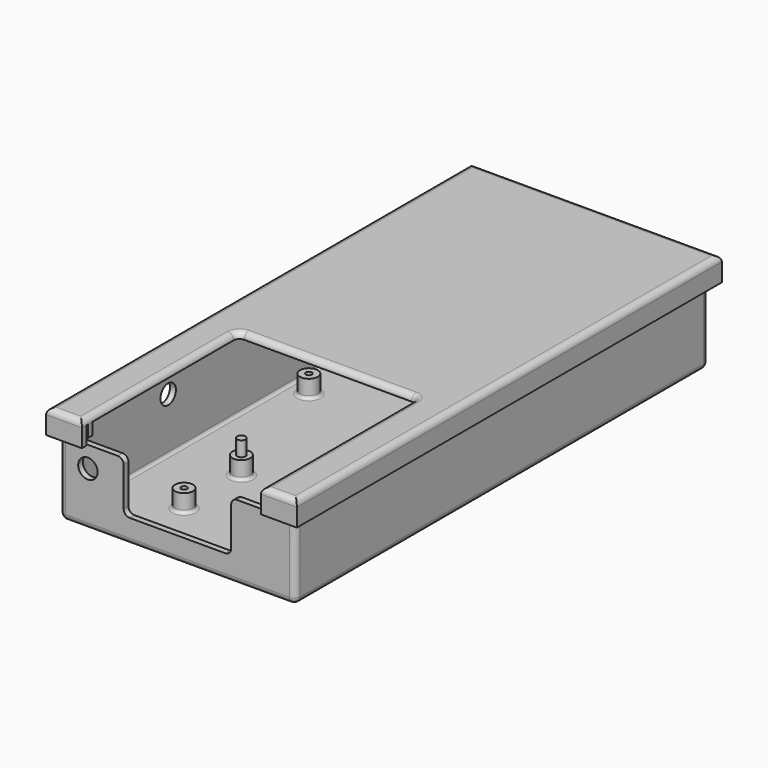
from build123d import *

# Parameters (mm, degrees)
F0_W      = 75
F0_H      = 169
F0_R      = 3
F1_DEPTH  = 2
F0_W_2    = 79
F0_H_2    = 173
F2_DEPTH  = 25
F3_DEPTH  = 8
F4_R      = 1.4
F5_DEPTH  = 5
F4_R_2    = 1
F6_DEPTH  = 6
F7_W      = 36
F7_H      = 17
F8_DEPTH  = 2
F10_R     = 2
F11_R     = 1
F12_R     = 2
F13_R     = 3.25
F14_DEPTH = 2
F15_R     = 3.25
F16_DEPTH = 2
F17_W     = 84
F17_H     = 178
F17_W_2   = 80
F17_H_2   = 174
F18_DEPTH = 8
F19_DEPTH = 6
F20_DEPTH = 2
F21_W     = 60
F21_H     = 65.5
F22_DEPTH = 8.001
F23_R     = 1.99999


# Not quite as in the source:
# - a fillet or chamfer is up to 0.001 mm smaller than in the source, because OpenCascade refuses the exact size


with BuildPart() as f1:
    # F0 (on Top) → F1 (new body)
    with BuildSketch(Plane.XY):
        with Locations((0, -1.5)):
            Rectangle(F0_W, F0_H)
        with Locations((-15.5, -65.85)):
            Circle(F0_R, mode=Mode.SUBTRACT)
        with Locations((-15.5, -41.85)):
            Circle(F0_R, mode=Mode.SUBTRACT)
        with Locations((15.5, -65.85)):
            Circle(F0_R, mode=Mode.SUBTRACT)
        with Locations((15.5, -41.85)):
            Circle(F0_R, mode=Mode.SUBTRACT)
        with Locations((-30.5, 5.15)):
            Circle(F0_R, mode=Mode.SUBTRACT)
        with Locations((-14.25, 75.5)):
            Circle(F0_R, mode=Mode.SUBTRACT)
        with Locations((30.5, 5.15)):
            Circle(F0_R, mode=Mode.SUBTRACT)
        with Locations((14.25, 75.5)):
            Circle(F0_R, mode=Mode.SUBTRACT)
    extrude(amount=F1_DEPTH)

    # F0 (on Top) → F2 (join)
    with BuildSketch(Plane.XY):
        with Locations((0, -1.5)):
            Rectangle(F0_W_2, F0_H_2)
        with Locations((0, -1.5)):
            Rectangle(F0_W, F0_H, mode=Mode.SUBTRACT)
    extrude(amount=F2_DEPTH)

    # F0 (on Top) → F3 (join)
    with BuildSketch(Plane.XY):
        with Locations((-14.25, 75.5)):
            Circle(F0_R)
        with Locations((14.25, 75.5)):
            Circle(F0_R)
        with Locations((30.5, 5.15)):
            Circle(F0_R)
        with Locations((-30.5, 5.15)):
            Circle(F0_R)
        with Locations((15.5, -41.85)):
            Circle(F0_R)
        with Locations((15.5, -65.85)):
            Circle(F0_R)
        with Locations((-15.5, -41.85)):
            Circle(F0_R)
        with Locations((-15.5, -65.85)):
            Circle(F0_R)
    extrude(amount=F3_DEPTH)

    # F4 (on face) → F5 (join)
    with BuildSketch(Plane.XY.offset(8)):
        with Locations((-14.25, 75.5)):
            Circle(F4_R)
        with Locations((30.5, 5.15)):
            Circle(F4_R)
        with Locations((-15.5, -41.85)):
            Circle(F4_R)
        with Locations((15.5, -65.85)):
            Circle(F4_R)
    extrude(amount=F5_DEPTH)

    # F4 (on face) → F6 (cut)
    with BuildSketch(Plane.XY.offset(8)):
        with Locations((14.25, 75.5)):
            Circle(F4_R_2)
        with Locations((-30.5, 5.15)):
            Circle(F4_R_2)
        with Locations((15.5, -41.85)):
            Circle(F4_R_2)
        with Locations((-15.5, -65.85)):
            Circle(F4_R_2)
    extrude(amount=-F6_DEPTH, mode=Mode.SUBTRACT)

    # F7 (on face) → F8 (cut, through all)
    with BuildSketch(Plane.XZ.offset(88)):
        with Locations((0, 16.5)):
            Rectangle(F7_W, F7_H)
    extrude(amount=-F8_DEPTH, mode=Mode.SUBTRACT)

    # F10
    f10_edges = [f1.edges().sort_by_distance(p)[0] for p in [
        (-39.5, -1.5, 0),
        (39.5, -1.5, 0),
        (0, -88, 0),
        (0, 85, 0),
        (37.5, 83, 13.5),
        (-37.5, 83, 13.5),
        (-37.5, -86, 13.5),
        (37.5, -86, 13.5),
        (39.5, -88, 12.5),
        (39.5, 85, 12.5),
        (-39.5, 85, 12.5),
        (-39.5, -88, 12.5),
    ]]
    fillet(f10_edges, radius=F10_R)

    # F11
    f11_edges = [f1.edges().sort_by_distance(p)[0] for p in [
        (-18.5, -41.85, 2),
        (-33.5, 5.15, 2),
        (-17.25, 75.5, 2),
        (11.25, 75.5, 2),
        (0, 83, 2),
        (36.914214, 82.414214, 2),
        (-36.914214, 82.414214, 2),
        (37.5, -1.5, 2),
        (-37.5, -1.5, 2),
        (36.914214, -85.414214, 2),
        (-36.914214, -85.414214, 2),
        (0, -86, 2),
        (-18.5, -65.85, 2),
        (12.5, -65.85, 2),
        (12.5, -41.85, 2),
        (27.5, 5.15, 2),
    ]]
    fillet(f11_edges, radius=F11_R)

    # F12
    f12_edges = [f1.edges().sort_by_distance(p)[0] for p in [
        (-18, -87, 8),
        (18, -87, 8),
        (18, -87, 25),
        (-18, -87, 25),
    ]]
    fillet(f12_edges, radius=F12_R)

    # F13 (on face) → F14 (cut, through all)
    with BuildSketch(Plane(origin=(-39.5, 0, 0), x_dir=(0, -1, 0), z_dir=(-1, 0, 0))):
        with Locations((0, 20)):
            Circle(F13_R)
        with Locations((45, 20)):
            Circle(F13_R)
    extrude(amount=-F14_DEPTH, mode=Mode.SUBTRACT)

    # F15 (on face) → F16 (cut, through all)
    with BuildSketch(Plane.XZ.offset(88)):
        with Locations((-30, 18)):
            Circle(F15_R)
    extrude(amount=-F16_DEPTH, mode=Mode.SUBTRACT)


with BuildPart() as f18:
    # F17 (on face) → F18 (new body)
    with BuildSketch(Plane.XY.offset(25)):
        with Locations((0, -1.5)):
            Rectangle(F17_W, F17_H)
        with Locations((0, -1.5)):
            Rectangle(F17_W_2, F17_H_2, mode=Mode.SUBTRACT)
        with Locations((0, -1.5)):
            Rectangle(F17_W_2, F17_H_2)
        with BuildLine():
            Line((37.5, -88), (20, -88))
            Line((20, -88), (20, -86))
            Line((20, -86), (35.5, -86))
            ThreePointArc((35.5, -86), (36.9142135624, -85.4142135624), (37.5, -84))
            Line((37.5, -84), (37.5, 81))
            ThreePointArc((37.5, 81), (36.9142135624, 82.4142135624), (35.5, 83))
            Line((35.5, 83), (-35.5, 83))
            ThreePointArc((-35.5, 83), (-36.9142135624, 82.4142135624), (-37.5, 81))
            Line((-37.5, 81), (-37.5, -84))
            ThreePointArc((-37.5, -84), (-36.9142135624, -85.4142135624), (-35.5, -86))
            Line((-35.5, -86), (-20, -86))
            Line((-20, -86), (-20, -88))
            Line((-20, -88), (-37.5, -88))
            ThreePointArc((-37.5, -88), (-38.9142135624, -87.4142135624), (-39.5, -86))
            Line((-39.5, -86), (-39.5, 83))
            ThreePointArc((-39.5, 83), (-38.9142135624, 84.4142135624), (-37.5, 85))
            Line((-37.5, 85), (37.5, 85))
            ThreePointArc((37.5, 85), (38.9142135624, 84.4142135624), (39.5, 83))
            Line((39.5, 83), (39.5, -86))
            ThreePointArc((39.5, -86), (38.9142135624, -87.4142135624), (37.5, -88))
        make_face(mode=Mode.SUBTRACT)
        with BuildLine():
            Line((20, -86), (20, -88))
            Line((20, -88), (37.5, -88))
            ThreePointArc((37.5, -88), (38.9142135624, -87.4142135624), (39.5, -86))
            Line((39.5, -86), (39.5, 83))
            ThreePointArc((39.5, 83), (38.9142135624, 84.4142135624), (37.5, 85))
            Line((37.5, 85), (-37.5, 85))
            ThreePointArc((-37.5, 85), (-38.9142135624, 84.4142135624), (-39.5, 83))
            Line((-39.5, 83), (-39.5, -86))
            ThreePointArc((-39.5, -86), (-38.9142135624, -87.4142135624), (-37.5, -88))
            Line((-37.5, -88), (-20, -88))
            Line((-20, -88), (-20, -86))
            Line((-20, -86), (-35.5, -86))
            ThreePointArc((-35.5, -86), (-36.9142135624, -85.4142135624), (-37.5, -84))
            Line((-37.5, -84), (-37.5, 81))
            ThreePointArc((-37.5, 81), (-36.9142135624, 82.4142135624), (-35.5, 83))
            Line((-35.5, 83), (35.5, 83))
            ThreePointArc((35.5, 83), (36.9142135624, 82.4142135624), (37.5, 81))
            Line((37.5, 81), (37.5, -84))
            ThreePointArc((37.5, -84), (36.9142135624, -85.4142135624), (35.5, -86))
            Line((35.5, -86), (20, -86))
        make_face()
    extrude(amount=F18_DEPTH)

    # F17 (on face) → F19 (cut)
    with BuildSketch(Plane.XY.offset(25)):
        with Locations((0, -1.5)):
            Rectangle(F17_W_2, F17_H_2)
        with BuildLine():
            Line((37.5, -88), (20, -88))
            Line((20, -88), (20, -86))
            Line((20, -86), (35.5, -86))
            ThreePointArc((35.5, -86), (36.9142135624, -85.4142135624), (37.5, -84))
            Line((37.5, -84), (37.5, 81))
            ThreePointArc((37.5, 81), (36.9142135624, 82.4142135624), (35.5, 83))
            Line((35.5, 83), (-35.5, 83))
            ThreePointArc((-35.5, 83), (-36.9142135624, 82.4142135624), (-37.5, 81))
            Line((-37.5, 81), (-37.5, -84))
            ThreePointArc((-37.5, -84), (-36.9142135624, -85.4142135624), (-35.5, -86))
            Line((-35.5, -86), (-20, -86))
            Line((-20, -86), (-20, -88))
            Line((-20, -88), (-37.5, -88))
            ThreePointArc((-37.5, -88), (-38.9142135624, -87.4142135624), (-39.5, -86))
            Line((-39.5, -86), (-39.5, 83))
            ThreePointArc((-39.5, 83), (-38.9142135624, 84.4142135624), (-37.5, 85))
            Line((-37.5, 85), (37.5, 85))
            ThreePointArc((37.5, 85), (38.9142135624, 84.4142135624), (39.5, 83))
            Line((39.5, 83), (39.5, -86))
            ThreePointArc((39.5, -86), (38.9142135624, -87.4142135624), (37.5, -88))
        make_face(mode=Mode.SUBTRACT)
    extrude(amount=F19_DEPTH, mode=Mode.SUBTRACT)

    # F17 (on face) → F20 (cut)
    with BuildSketch(Plane.XY.offset(25)):
        with BuildLine():
            Line((20, -86), (20, -88))
            Line((20, -88), (37.5, -88))
            ThreePointArc((37.5, -88), (38.9142135624, -87.4142135624), (39.5, -86))
            Line((39.5, -86), (39.5, 83))
            ThreePointArc((39.5, 83), (38.9142135624, 84.4142135624), (37.5, 85))
            Line((37.5, 85), (-37.5, 85))
            ThreePointArc((-37.5, 85), (-38.9142135624, 84.4142135624), (-39.5, 83))
            Line((-39.5, 83), (-39.5, -86))
            ThreePointArc((-39.5, -86), (-38.9142135624, -87.4142135624), (-37.5, -88))
            Line((-37.5, -88), (-20, -88))
            Line((-20, -88), (-20, -86))
            Line((-20, -86), (-35.5, -86))
            ThreePointArc((-35.5, -86), (-36.9142135624, -85.4142135624), (-37.5, -84))
            Line((-37.5, -84), (-37.5, 81))
            ThreePointArc((-37.5, 81), (-36.9142135624, 82.4142135624), (-35.5, 83))
            Line((-35.5, 83), (35.5, 83))
            ThreePointArc((35.5, 83), (36.9142135624, 82.4142135624), (37.5, 81))
            Line((37.5, 81), (37.5, -84))
            ThreePointArc((37.5, -84), (36.9142135624, -85.4142135624), (35.5, -86))
            Line((35.5, -86), (20, -86))
        make_face()
    extrude(amount=F20_DEPTH, mode=Mode.SUBTRACT)

    # F21 (on face) → F22 (cut, through all)
    with BuildSketch(Plane.XY.offset(33)):
        with Locations((0, -57.75)):
            Rectangle(F21_W, F21_H)
    extrude(amount=-F22_DEPTH, mode=Mode.SUBTRACT)

    # F23 (radius 2 in the source; OpenCascade refuses exactly that, so slightly less here)
    f23_edges = [f18.edges().sort_by_distance(p)[0] for p in [
        (-42, -1.5, 33),
        (42, -1.5, 33),
        (36, -90.5, 33),
        (-36, -90.5, 33),
        (0, 87.5, 33),
        (-30, -25, 32),
        (30, -25, 32),
        (-30, -57.75, 33),
        (30, -57.75, 33),
        (0, -25, 33),
    ]]
    fillet(f23_edges, radius=F23_R)


solid = Compound([f1.part, f18.part])
